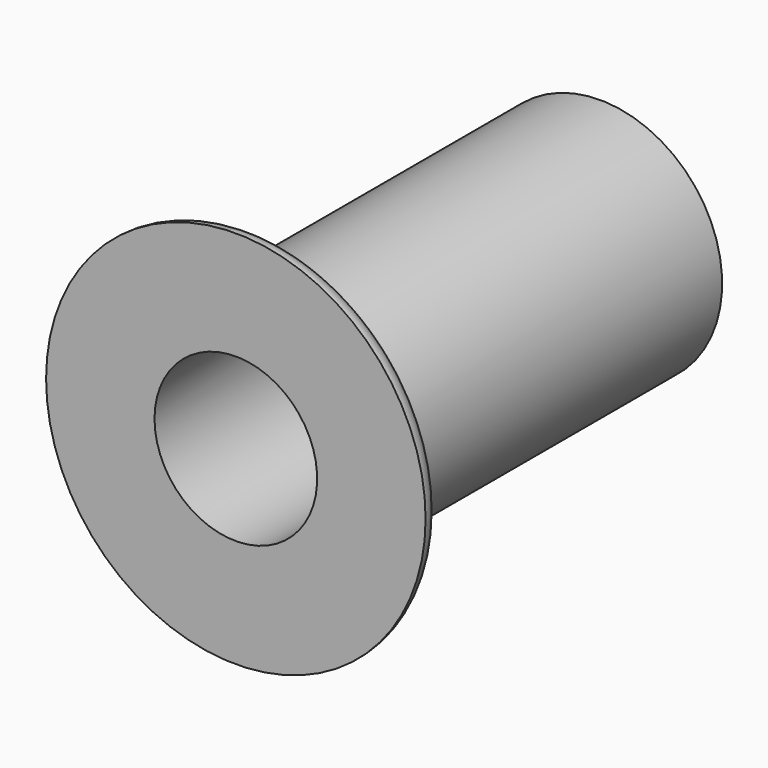
from build123d import *

# Parameters (mm, degrees)
F0_R     = 44.45
F1_DEPTH = 5.08
F2_R     = 5.07999
F4_R     = 28.575
F5_DEPTH = 101.6
F6_D     = 38.1
F6_DEPTH = 38.1
F6_TIP   = 11.4463947925


# Not quite as in the source:
# - a fillet or chamfer is up to 0.001 mm smaller than in the source, because OpenCascade refuses the exact size


with BuildPart() as f1:
    # F0 (on Front) → F1 (new body)
    with BuildSketch(Plane.XZ):
        Circle(F0_R)
    extrude(amount=F1_DEPTH)

    # F2 (radius 5.08 in the source; OpenCascade refuses exactly that, so slightly less here)
    f2_edges = [f1.edges().sort_by_distance(p)[0] for p in [
        (-44.45, 0, 0),
    ]]
    fillet(f2_edges, radius=F2_R)

    # F4 (on face) → F5 (join)
    with BuildSketch(Plane(origin=(0, 0, 0), x_dir=(-1, 0, 0), z_dir=(0, 1, 0))):
        Circle(F4_R)
    extrude(amount=F5_DEPTH)

    # F6
    with Locations(Plane.XZ.offset(5.08)):
        with Locations((0, 0)):
            Hole(F6_D / 2, depth=F6_DEPTH)
            with Locations((0, 0, -(F6_DEPTH + F6_TIP / 2))):  # 118° drill point
                Cone(0, F6_D / 2, F6_TIP, mode=Mode.SUBTRACT)


solid = f1.part
